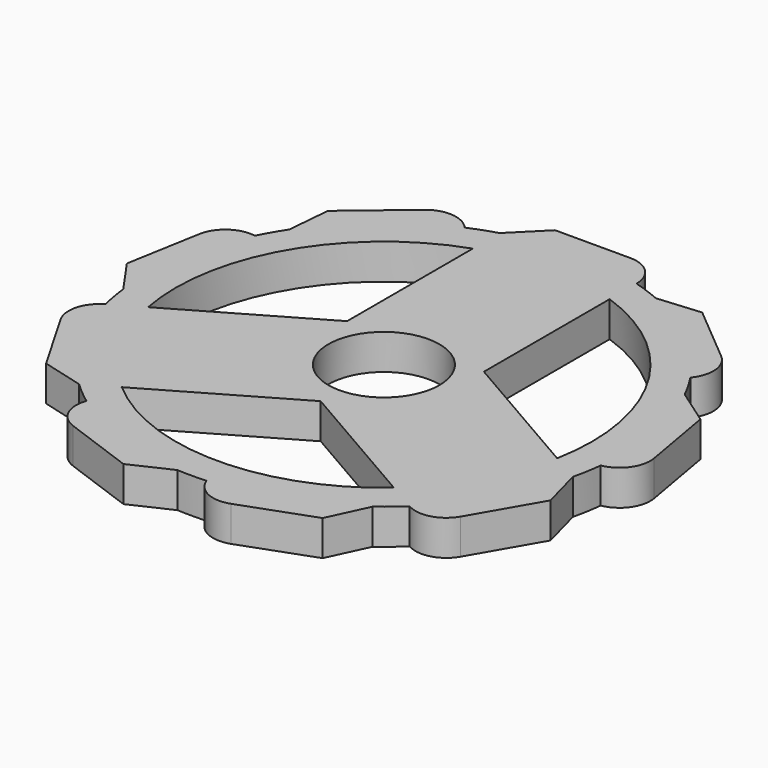
from build123d import *

# Parameters (mm, degrees)
F0_R     = 13.5636
F0_R_2   = 11
F1_DEPTH = 7


# Not quite as in the source:
# - a feature names something its author has since deleted; it is built from what else it names


with BuildPart() as f1:
    # F0 (on Top) → F1 (new body)
    with BuildSketch(Plane.XY):
        with BuildLine():
            Line((-7.4638039729, 51.7525), (-13.5636, 45.6527039729))
            ThreePointArc((-13.5636, 45.6527039729), (-16.2887093259, 44.7528610649), (-18.9546720538, 43.6905142146))
            ThreePointArc((-18.9546720538, 43.6905142146), (-23.0957546511, 45.8462253684), (-27.5482602123, 44.4423557574))
            Line((-27.5482602123, 44.4423557574), (-38.9834713283, 34.8470743276))
            Line((-38.9834713283, 34.8470743276), (-39.7353128712, 26.2534861691))
            ThreePointArc((-39.7353128712, 26.2534861691), (-41.2444598552, 23.8125), (-42.6038423959, 21.2850472892))
            ThreePointArc((-42.6038423959, 21.2850472892), (-47.1617601278, 20.2745812553), (-49.6701872794, 16.3371393342))
            Line((-49.6701872794, 16.3371393342), (-52.2623391961, 1.6363152952))
            Line((-52.2623391961, 1.6363152952), (-47.3144312411, -5.4300295883))
            ThreePointArc((-47.3144312411, -5.4300295883), (-46.9014692372, -8.2699944614), (-46.318201392, -11.0799298197))
            ThreePointArc((-46.318201392, -11.0799298197), (-49.1602538961, -14.783764754), (-48.5508816958, -19.4124061506))
            Line((-48.5508816958, -19.4124061506), (-41.0870777229, -32.3400938494))
            Line((-41.0870777229, -32.3400938494), (-32.754601392, -34.5727741532))
            ThreePointArc((-32.754601392, -34.5727741532), (-30.6127599113, -36.4828666035), (-28.3597591873, -38.2604846263))
            ThreePointArc((-28.3597591873, -38.2604846263), (-28.156118511, -42.9246229316), (-24.7140789838, -46.0786710526))
            Line((-24.7140789838, -46.0786710526), (-10.6867159511, -51.1842136618))
            Line((-10.6867159511, -51.1842136618), (-2.8685295247, -47.5385334583))
            ThreePointArc((-2.8685295247, -47.5385334583), (0, -47.625), (2.8685295247, -47.5385334583))
            ThreePointArc((2.8685295247, -47.5385334583), (6.0225776457, -50.9805729855), (10.6867159511, -51.1842136618))
            Line((10.6867159511, -51.1842136618), (24.7140789838, -46.0786710526))
            Line((24.7140789838, -46.0786710526), (28.3597591873, -38.2604846263))
            ThreePointArc((28.3597591873, -38.2604846263), (30.6127599113, -36.4828666035), (32.754601392, -34.5727741532))
            ThreePointArc((32.754601392, -34.5727741532), (37.3832427886, -35.1821463535), (41.0870777229, -32.3400938494))
            Line((41.0870777229, -32.3400938494), (48.5508816958, -19.4124061506))
            Line((48.5508816958, -19.4124061506), (46.318201392, -11.0799298197))
            ThreePointArc((46.318201392, -11.0799298197), (46.9014692372, -8.2699944614), (47.3144312411, -5.4300295883))
            ThreePointArc((47.3144312411, -5.4300295883), (51.2518731622, -2.9216024367), (52.2623391961, 1.6363152952))
            Line((52.2623391961, 1.6363152952), (49.6701872794, 16.3371393342))
            Line((49.6701872794, 16.3371393342), (42.6038423959, 21.2850472892))
            ThreePointArc((42.6038423959, 21.2850472892), (41.2444598552, 23.8125), (39.7353128712, 26.2534861691))
            ThreePointArc((39.7353128712, 26.2534861691), (41.1391824821, 30.7059917302), (38.9834713283, 34.8470743276))
            Line((38.9834713283, 34.8470743276), (27.5482602123, 44.4423557574))
            Line((27.5482602123, 44.4423557574), (18.9546720538, 43.6905142146))
            ThreePointArc((18.9546720538, 43.6905142146), (16.2887093259, 44.7528610649), (13.5636, 45.6527039729))
            ThreePointArc((13.5636, 45.6527039729), (11.7770111075, 49.9659111075), (7.4638039729, 51.7525))
            Line((7.4638039729, 51.7525), (-7.4638039729, 51.7525))
        make_face()
        with BuildLine():
            ThreePointArc((26.9782471716, -31.2377944892), (0, -41.275), (-26.9782471716, -31.2377944892))
            Line((-26.9782471716, -31.2377944892), (0, -15.6618962224))
            Line((0, -15.6618962224), (26.9782471716, -31.2377944892))
        make_face(mode=Mode.SUBTRACT)
        Circle(F0_R, mode=Mode.SUBTRACT)
        with BuildLine():
            ThreePointArc((-40.5418471716, -7.7449501556), (-35.7451985412, 20.6375), (-13.5636, 38.9827446448))
            Line((-13.5636, 38.9827446448), (-13.5636, 7.8309481112))
            Line((-13.5636, 7.8309481112), (-40.5418471716, -7.7449501556))
        make_face(mode=Mode.SUBTRACT)
        with BuildLine():
            ThreePointArc((13.5636, 38.9827446448), (35.7451985412, 20.6375), (40.5418471716, -7.7449501556))
            Line((40.5418471716, -7.7449501556), (13.5636, 7.8309481112))
            Line((13.5636, 7.8309481112), (13.5636, 38.9827446448))
        make_face(mode=Mode.SUBTRACT)
        Circle(F0_R)
        Circle(F0_R_2, mode=Mode.SUBTRACT)
    extrude(amount=F1_DEPTH)


solid = f1.part
